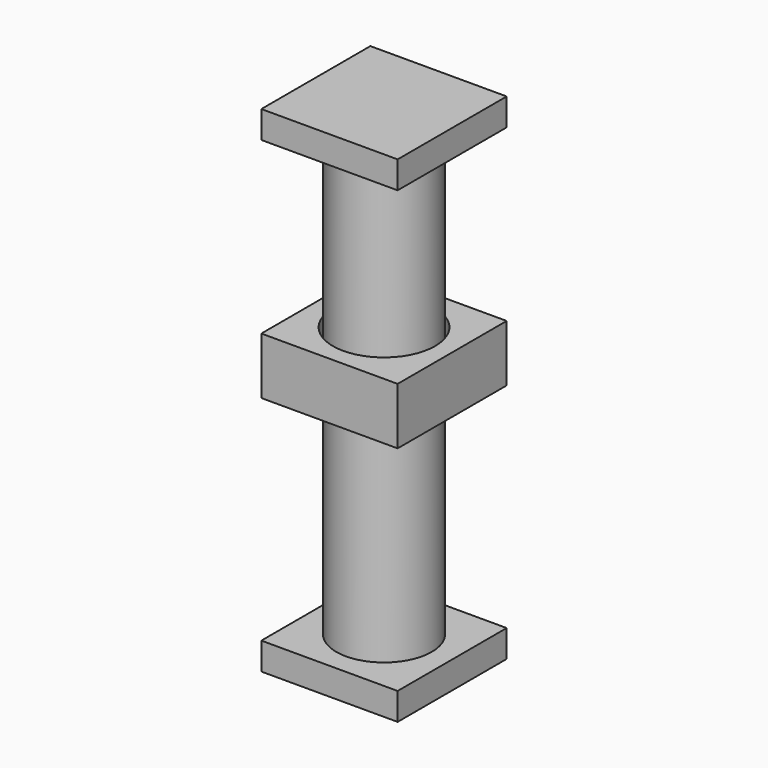
from build123d import *

# Parameters (mm, degrees)
F0_W     = 60
F0_H     = 60
F1_DEPTH = 25
F2_R     = 22.5
F3_DEPTH = 25.001
F4_R     = 21
F5_DEPTH = 100
F7_W     = 60
F7_H     = 60
F7_R     = 21
F8_DEPTH = 6
F6_W     = 60
F6_H     = 60
F9_DEPTH = 12


with BuildPart() as f1:
    # F0 (on Top) → F1 (new body)
    with BuildSketch(Plane.XY):
        Rectangle(F0_W, F0_H)
    extrude(amount=F1_DEPTH)

    # F2 (on face) → F3 (cut, through all)
    with BuildSketch(Plane.XY.offset(25)):
        Circle(F2_R)
    extrude(amount=-F3_DEPTH, mode=Mode.SUBTRACT)


with BuildPart() as f5:
    # F4 (on Top) → F5 (new body, symmetric)
    with BuildSketch(Plane.XY):
        Circle(F4_R)
    extrude(amount=F5_DEPTH, both=True)

    # F7 (on face) → F8 (join, symmetric)
    with BuildSketch(Plane(origin=(0, 0, -100), x_dir=(1, 0, 0), z_dir=(0, 0, -1))):
        Rectangle(F7_W, F7_H)
        Circle(F7_R, mode=Mode.SUBTRACT)
        Circle(F7_R)
    extrude(amount=F8_DEPTH, both=True)

    # F6 (on face) → F9 (join)
    with BuildSketch(Plane.XY.offset(100)):
        Rectangle(F6_W, F6_H)
    extrude(amount=F9_DEPTH)


solid = Compound([f1.part, f5.part])
